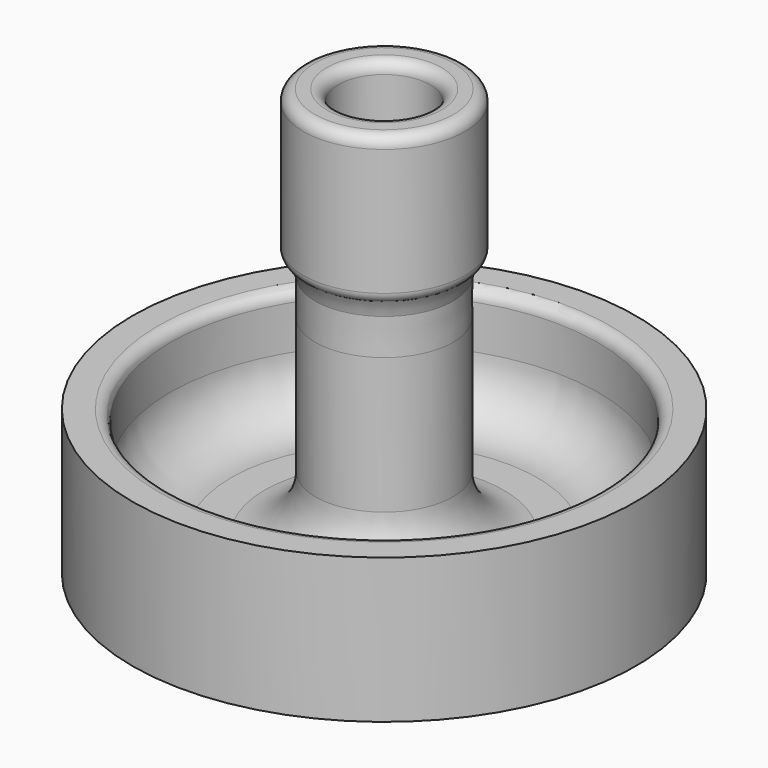
from build123d import *

# Parameters (mm, degrees)
F3_R = 0.5


# Not quite as in the source:
# - a fillet or chamfer that OpenCascade refuses, or shapes differently, is made with other operations: its cross-section is extruded or revolved along the edge and cut away or added
# - a feature names something its author has since deleted; it is built from what else it names


with BuildPart() as f1:
    # F0 (on Front) → F1 (revolve)
    with BuildSketch(Plane.XZ):
        with BuildLine():
            Line((-11.0497801401, 0), (-6.35, 0))
            ThreePointArc((-6.35, 0), (-3.6810616685, -0.5842717783), (-1.5003500059, -2.2302067626))
            ThreePointArc((-1.5003500059, -2.2302067626), (-1.292996294, -0.7904112116), (0, -0.1239523798))
            Line((0, -0.1239523798), (0, 0))
            Line((0, 0), (0, 4.6583339572))
            Line((0, 4.6583339572), (-1.5205304027, 4.6583339572))
            ThreePointArc((-1.5205304027, 4.6583339572), (-1.8740837933, 4.8047805666), (-2.0205304027, 5.1583339572))
            Line((-2.0205304027, 5.1583339572), (-2.0205304027, 18.7134853154))
            Line((-2.0205304027, 18.7134853154), (-3.0250614509, 18.7134853154))
            Line((-3.0250614509, 18.7134853154), (-3.5481122322, 18.7134853154))
            Line((-3.5481122322, 18.7134853154), (-3.5481122322, 12.2134853154))
            Line((-3.5481122322, 12.2134853154), (-3.2865868416, 12.2134853154))
            ThreePointArc((-3.2865868416, 12.2134853154), (-3.1265563478, 11.8601003085), (-3.0236392793, 11.4860698297))
            Line((-3.0236392793, 11.4860698297), (-3.0205304027, 9.8959347233))
            Line((-3.0205304027, 9.8959347233), (-3.0205304027, 3.925))
            ThreePointArc((-3.0205304027, 3.925), (-3.6626216951, 2.2779224085), (-5.2500669844, 1.5))
            Line((-5.2500669844, 1.5), (-6.7232404836, 1.5))
            ThreePointArc((-6.7232404836, 1.5), (-8.5932958155, 2.1254805036), (-9.3995602801, 3.925))
            Line((-9.3995602801, 3.925), (-9.3995602801, 5.85))
            ThreePointArc((-9.3995602801, 5.85), (-9.5460068896, 6.2035533906), (-9.8995602801, 6.35))
            Line((-9.8995602801, 6.35), (-11.0497801401, 6.35))
            Line((-11.0497801401, 6.35), (-11.0497801401, 0))
        make_face()
    revolve(axis=Axis((0, 0, 3.175), (0, 0, 1)))

    # F2: fillet of radius 0.5 on 2 edges, made by hand

    # F2_s1 → F2_t2 (revolve, cut)
    with BuildSketch(Plane.XZ):
        with BuildLine():
            ThreePointArc((-3.0481122322, 18.7134853154), (-3.4016656228, 18.567038706), (-3.5481122322, 18.2134853154))
            Line((-3.5481122322, 18.2134853154), (-3.5581122322, 18.2134853154))
            Line((-3.5581122322, 18.2134853154), (-3.5581122322, 18.7234853154))
            Line((-3.5581122322, 18.7234853154), (-3.0481122322, 18.7234853154))
            Line((-3.0481122322, 18.7234853154), (-3.0481122322, 18.7134853154))
        make_face()
    revolve(axis=Axis((0, 0, 18.7134853154), (0, 0, 1)), mode=Mode.SUBTRACT)

    # F2_s3 → F2_t4 (revolve, cut)
    with BuildSketch(Plane.XZ):
        with BuildLine():
            ThreePointArc((-3.2865868416, 12.2134853154), (-3.4777849592, 12.3972529753), (-3.5481122322, 12.6529507415))
            Line((-3.5481122322, 12.6529507415), (-3.5581122322, 12.6529507415))
            Line((-3.5581122322, 12.6529507415), (-3.5581122322, 12.2134853154))
            Line((-3.5581122322, 12.2134853154), (-3.5481122322, 12.2034853154))
            ThreePointArc((-3.5481122322, 12.2034853154), (-3.4173495369, 12.2034853154), (-3.2913563338, 12.2046960069))
            Line((-3.2913563338, 12.2046960069), (-3.2865868416, 12.2134853154))
        make_face()
    revolve(axis=Axis((0, 0, 12.2134853154), (0, 0, 1)), mode=Mode.SUBTRACT)

    # F3
    f3_edges = [f1.edges().sort_by_distance(p)[0] for p in [
        (2.02053, 0, 18.713485),
    ]]
    fillet(f3_edges, radius=F3_R)


solid = f1.part
